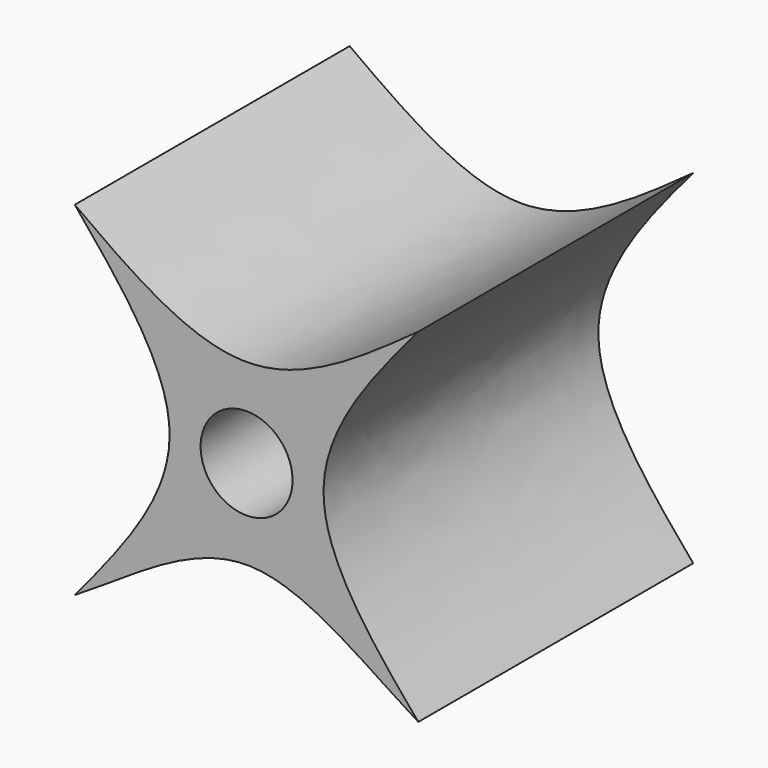
from build123d import *

# Parameters (mm, degrees)
F0_W     = 25.4
F0_H     = 25.4
F1_DEPTH = 25.4
F3_DEPTH = 25.401
F4_DEPTH = 25.4010001
F5_DEPTH = 25.4010001
F6_DEPTH = 25.4010001
F7_R     = 3.3987951376
F8_DEPTH = 25.4010001


with BuildPart() as f1:
    # F0 (on Front) → F1 (new body)
    with BuildSketch(Plane.XZ):
        Rectangle(F0_W, F0_H)
    extrude(amount=F1_DEPTH)

    # F2 (on face) → F3 (cut, through all)
    with BuildSketch(Plane.XZ.offset(25.4)):
        with BuildLine():
            add(Edge.make_bspline(
                [(-12.7, 12.7), (-9.1949671809, 8.4666666667), (-2.1849015426, 0), (-9.1949671809, -8.4666666667), (-12.7, -12.7)],
                knots=[0, 0, 0, 0, 0.5, 1, 1, 1, 1], degree=3))
            Line((-12.7, 12.7), (-12.7, -12.7))
        make_face()
    extrude(amount=-F3_DEPTH, mode=Mode.SUBTRACT)

    # F2 (on face) → F4 (cut, through all)
    with BuildSketch(Plane.XZ.offset(25.4)):
        with BuildLine():
            Line((12.7, 12.7), (-12.7, 12.7))
            add(Edge.make_bspline(
                [(-12.7, 12.7), (-8.4666666667, 9.6461512916), (0, 3.5384538747), (8.4666666667, 9.6461512916), (12.7, 12.7)],
                knots=[0, 0, 0, 0, 0.5, 1, 1, 1, 1], degree=3))
        make_face()
    extrude(amount=-F4_DEPTH, mode=Mode.SUBTRACT)

    # F2 (on face) → F5 (cut, through all)
    with BuildSketch(Plane.XZ.offset(25.4)):
        with BuildLine():
            Line((12.7, -12.7), (12.7, 12.7))
            add(Edge.make_bspline(
                [(12.7, 12.7), (9.0947037864, 8.4666666667), (2.2844962136, 0), (9.0947037864, -8.4666666667), (12.7, -12.7)],
                knots=[0, 0, 0, 0, 0.5, 1, 1, 1, 1], degree=3))
        make_face()
    extrude(amount=-F5_DEPTH, mode=Mode.SUBTRACT)

    # F2 (on face) → F6 (cut, through all)
    with BuildSketch(Plane.XZ.offset(25.4)):
        with BuildLine():
            add(Edge.make_bspline(
                [(-12.7, -12.7), (-8.4666666667, -10.1224012509), (0, -3.0855987491), (8.4666666667, -10.1224012509), (12.7, -12.7)],
                knots=[0, 0, 0, 0, 0.5, 1, 1, 1, 1], degree=3))
            Line((-12.7, -12.7), (12.7, -12.7))
        make_face()
    extrude(amount=-F6_DEPTH, mode=Mode.SUBTRACT)

    # F7 (on face) → F8 (cut, through all)
    with BuildSketch(Plane.XZ.offset(25.4)):
        Circle(F7_R)
    extrude(amount=-F8_DEPTH, mode=Mode.SUBTRACT)


solid = f1.part
